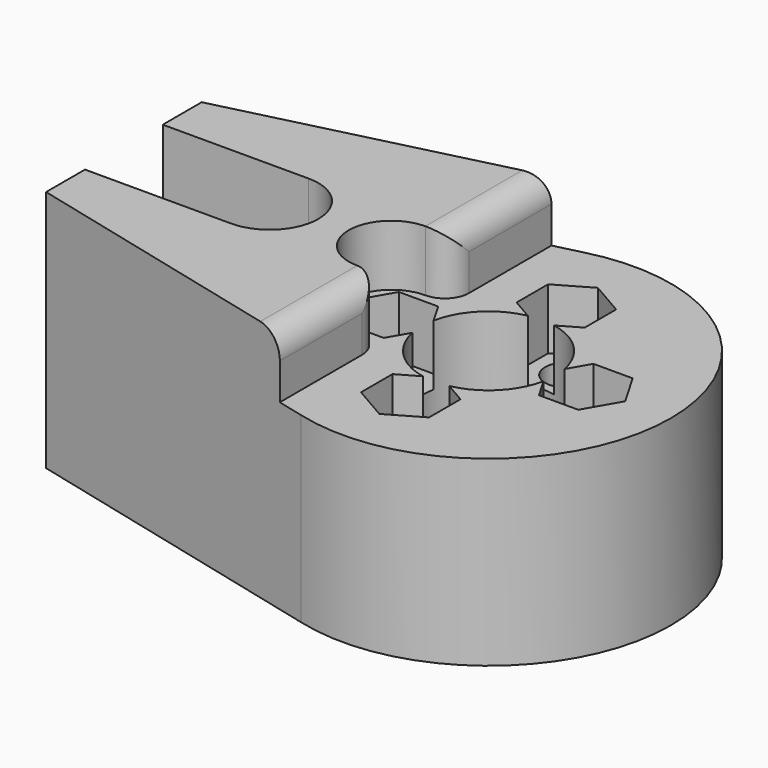
from build123d import *

# Parameters (mm, degrees)
F0_R     = 5.5
F1_DEPTH = 20
F3_D     = 3.5
F5_DEPTH = 10
F7_DEPTH = 5
F8_R     = 1.99999


# Not quite as in the source:
# - a fillet or chamfer is up to 0.001 mm smaller than in the source, because OpenCascade refuses the exact size


with BuildPart() as f1:
    # F0 (on Top) → F1 (new body)
    with BuildSketch(Plane.XY):
        with BuildLine():
            ThreePointArc((-18, 4), (-14, 0), (-18, -4))
            Line((-18, -4), (-30, -4))
            Line((-30, -4), (-30, -8))
            Line((-30, -8), (-3.8358095935, -14.5012607991))
            ThreePointArc((-3.8358095935, -14.5012607991), (15, 0), (-3.8358095935, 14.5012607991))
            Line((-3.8358095935, 14.5012607991), (-30, 8))
            Line((-30, 8), (-30, 4))
            Line((-30, 4), (-18, 4))
        make_face()
        Circle(F0_R, mode=Mode.SUBTRACT)
    extrude(amount=F1_DEPTH)

    # F3 (through all)
    with Locations(Plane.XY.offset(20)):
        with Locations((8, 0), (0, -8), (-8, 0), (0, 8)):
            Hole(F3_D / 2)

    # F4 (on face) → F5 (cut)
    with BuildSketch(Plane.XY.offset(20)):
        Polygon((11.2331615075, 0), (9.6165807537, 2.8), (6.3834192463, 2.8), (4.7668384925, 0), (6.3834192463, -2.8), (9.6165807537, -2.8), align=None)
        Polygon((-2.8, 9.6165807537), (-2.8, 6.3834192463), (0, 4.7668384925), (2.8, 6.3834192463), (2.8, 9.6165807537), (0, 11.2331615075), align=None)
        Polygon((-9.6165807537, -2.8), (-6.3834192463, -2.8), (-4.7668384925, 0), (-6.3834192463, 2.8), (-9.6165807537, 2.8), (-11.2331615075, 0), align=None)
        Polygon((2.8, -9.6165807537), (2.8, -6.3834192463), (0, -4.7668384925), (-2.8, -6.3834192463), (-2.8, -9.6165807537), (0, -11.2331615075), align=None)
    extrude(amount=-F5_DEPTH, mode=Mode.SUBTRACT)

    # F6 (on face) → F7 (cut)
    with BuildSketch(Plane.XY.offset(20)):
        with BuildLine():
            Line((-6, -13.9635041923), (-3.8358095935, -14.5012607991))
            ThreePointArc((-3.8358095935, -14.5012607991), (15, 0), (-3.8358095935, 14.5012607991))
            Line((-3.8358095935, 14.5012607991), (-6, 13.9635041923))
            Line((-6, 13.9635041923), (-6, 3.5))
            Line((-6, 3.5), (-8, 3.5))
            ThreePointArc((-8, 3.5), (-11.5, 0), (-8, -3.5))
            Line((-8, -3.5), (-6, -3.5))
            Line((-6, -3.5), (-6, -13.9635041923))
        make_face()
    extrude(amount=-F7_DEPTH, mode=Mode.SUBTRACT)

    # F8 (radius 2 in the source; OpenCascade refuses exactly that, so slightly less here)
    f8_edges = [f1.edges().sort_by_distance(p)[0] for p in [
        (-6, -8.731752, 20),
        (-6, 8.731752, 20),
        (-6, -3.5, 17.5),
        (-6, 3.5, 17.5),
    ]]
    fillet(f8_edges, radius=F8_R)


solid = f1.part
